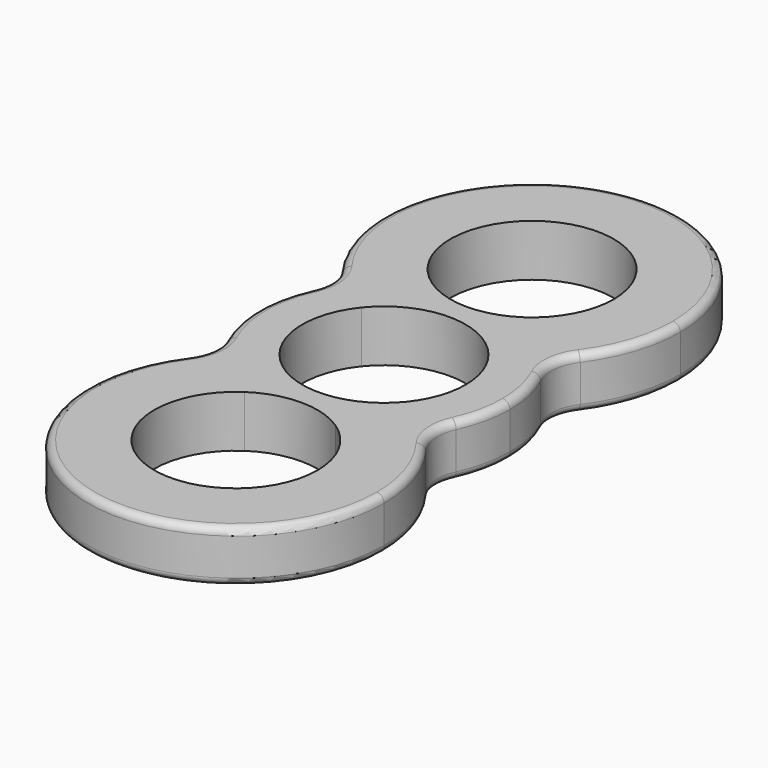
from build123d import *

# Parameters (mm, degrees)
F1_DEPTH = 7
F2_R     = 1


# Not quite as in the source:
# - a feature names something its author has since deleted; it is built from what else it names


with BuildPart() as f1:
    # F0 (on Top) → F1 (new body)
    with BuildSketch(Plane.XY):
        with BuildLine():
            ThreePointArc((8.5900351571, 6.911), (10.3984557172, 3.6637062787), (11.025, 0))
            ThreePointArc((11.025, 0), (10.3984557172, -3.6637062787), (8.5900351571, -6.911))
            ThreePointArc((8.5900351571, -6.911), (11.2087291798, -8.4058740762), (13.5732787491, -10.277))
            ThreePointArc((13.5732787491, -10.277), (14.5991765239, -8.7586911022), (15.455952476, -7.1389185498))
            ThreePointArc((15.455952476, -7.1389185498), (16.628111978, -3.6546568989), (17.025, 0))
            ThreePointArc((17.025, 0), (16.628111978, 3.6546568989), (15.455952476, 7.1389185498))
            ThreePointArc((15.455952476, 7.1389185498), (14.5991765239, 8.7586911022), (13.5732787491, 10.277))
            ThreePointArc((13.5732787491, 10.277), (11.2087291798, 8.4058740762), (8.5900351571, 6.911))
        make_face()
        with BuildLine():
            ThreePointArc((-8.5900351571, -6.911), (-11.025, 0), (-8.5900351571, 6.911))
            ThreePointArc((-8.5900351571, 6.911), (-11.2087291798, 8.4058740762), (-13.5732787491, 10.277))
            ThreePointArc((-13.5732787491, 10.277), (-14.5991765239, 8.7586911022), (-15.455952476, 7.1389185498))
            ThreePointArc((-15.455952476, 7.1389185498), (-17.025, 0), (-15.455952476, -7.1389185498))
            ThreePointArc((-15.455952476, -7.1389185498), (-14.5991765239, -8.7586911022), (-13.5732787491, -10.277))
            ThreePointArc((-13.5732787491, -10.277), (-11.2087291798, -8.4058740762), (-8.5900351571, -6.911))
        make_face()
        with BuildLine():
            ThreePointArc((6.1741937935, 15.866), (10.2615738659, 13.584944858), (13.5732787491, 10.277))
            ThreePointArc((13.5732787491, 10.277), (14.88595909, 11.6056412259), (16.0691422874, 13.0508037447))
            ThreePointArc((16.0691422874, 13.0508037447), (19.0103287623, 18.7065092876), (20.025, 25))
            ThreePointArc((20.025, 25), (-6.2934907124, 44.0103287623), (-16.0691422874, 13.0508037447))
            ThreePointArc((-16.0691422874, 13.0508037447), (-14.88595909, 11.6056412259), (-13.5732787491, 10.277))
            ThreePointArc((-13.5732787491, 10.277), (-10.2615738659, 13.584944858), (-6.1741937935, 15.866))
            ThreePointArc((-6.1741937935, 15.866), (-5.1710800819, 34.737071212), (11.025, 25))
            ThreePointArc((11.025, 25), (9.737071212, 19.8289199181), (6.1741937935, 15.866))
        make_face()
        with BuildLine():
            ThreePointArc((16.0691422874, 13.0508037447), (14.88595909, 11.6056412259), (13.5732787491, 10.277))
            ThreePointArc((13.5732787491, 10.277), (14.5991765239, 8.7586911022), (15.455952476, 7.1389185498))
            ThreePointArc((15.455952476, 7.1389185498), (14.9507513772, 10.1790618755), (16.0691422874, 13.0508037447))
        make_face()
        with BuildLine():
            ThreePointArc((16.0691422874, -13.0508037447), (14.88595909, -11.6056412259), (13.5732787491, -10.277))
            ThreePointArc((13.5732787491, -10.277), (10.2615738659, -13.584944858), (6.1741937935, -15.866))
            ThreePointArc((6.1741937935, -15.866), (9.737071212, -19.8289199181), (11.025, -25))
            ThreePointArc((11.025, -25), (-5.1710800819, -34.737071212), (-6.1741937935, -15.866))
            ThreePointArc((-6.1741937935, -15.866), (-10.2615738659, -13.584944858), (-13.5732787491, -10.277))
            ThreePointArc((-13.5732787491, -10.277), (-14.88595909, -11.6056412259), (-16.0691422874, -13.0508037447))
            ThreePointArc((-16.0691422874, -13.0508037447), (-6.2934907124, -44.0103287623), (20.025, -25))
            ThreePointArc((20.025, -25), (19.0103287623, -18.7065092876), (16.0691422874, -13.0508037447))
        make_face()
        with BuildLine():
            ThreePointArc((15.455952476, -7.1389185498), (14.5991765239, -8.7586911022), (13.5732787491, -10.277))
            ThreePointArc((13.5732787491, -10.277), (14.88595909, -11.6056412259), (16.0691422874, -13.0508037447))
            ThreePointArc((16.0691422874, -13.0508037447), (14.9507513772, -10.1790618755), (15.455952476, -7.1389185498))
        make_face()
        with BuildLine():
            ThreePointArc((-15.455952476, 7.1389185498), (-14.5991765239, 8.7586911022), (-13.5732787491, 10.277))
            ThreePointArc((-13.5732787491, 10.277), (-14.88595909, 11.6056412259), (-16.0691422874, 13.0508037447))
            ThreePointArc((-16.0691422874, 13.0508037447), (-14.9507513772, 10.1790618755), (-15.455952476, 7.1389185498))
        make_face()
        with BuildLine():
            ThreePointArc((-16.0691422874, -13.0508037447), (-14.88595909, -11.6056412259), (-13.5732787491, -10.277))
            ThreePointArc((-13.5732787491, -10.277), (-14.5991765239, -8.7586911022), (-15.455952476, -7.1389185498))
            ThreePointArc((-15.455952476, -7.1389185498), (-14.9507513772, -10.1790618755), (-16.0691422874, -13.0508037447))
        make_face()
        with BuildLine():
            ThreePointArc((-8.5900351571, 6.911), (0, 11.025), (8.5900351571, 6.911))
            ThreePointArc((8.5900351571, 6.911), (11.2087291798, 8.4058740762), (13.5732787491, 10.277))
            ThreePointArc((13.5732787491, 10.277), (10.2615738659, 13.584944858), (6.1741937935, 15.866))
            ThreePointArc((6.1741937935, 15.866), (0, 13.975), (-6.1741937935, 15.866))
            ThreePointArc((-6.1741937935, 15.866), (-10.2615738659, 13.584944858), (-13.5732787491, 10.277))
            ThreePointArc((-13.5732787491, 10.277), (-11.2087291798, 8.4058740762), (-8.5900351571, 6.911))
        make_face()
        with BuildLine():
            ThreePointArc((13.5732787491, -10.277), (11.2087291798, -8.4058740762), (8.5900351571, -6.911))
            ThreePointArc((8.5900351571, -6.911), (0, -11.025), (-8.5900351571, -6.911))
            ThreePointArc((-8.5900351571, -6.911), (-11.2087291798, -8.4058740762), (-13.5732787491, -10.277))
            ThreePointArc((-13.5732787491, -10.277), (-10.2615738659, -13.584944858), (-6.1741937935, -15.866))
            ThreePointArc((-6.1741937935, -15.866), (0, -13.975), (6.1741937935, -15.866))
            ThreePointArc((6.1741937935, -15.866), (10.2615738659, -13.584944858), (13.5732787491, -10.277))
        make_face()
    extrude(amount=F1_DEPTH)

    # F2
    f2_edges = [f1.edges().sort_by_distance(p)[0] for p in [
        (16.069142, 13.050804, 3.5),
        (-16.069142, 13.050804, 3.5),
        (0, 45.025, 0),
        (0, 45.025, 7),
        (-15.455952, 7.138919, 3.5),
        (-14.950751, 10.179062, 0),
        (-14.950751, 10.179062, 7),
        (-15.455952, -7.138919, 3.5),
        (-16.069142, -13.050804, 3.5),
        (-14.950751, -10.179062, 0),
        (-14.950751, -10.179062, 7),
        (16.069142, -13.050804, 3.5),
        (0, -45.025, 0),
        (0, -45.025, 7),
    ]]
    fillet(f2_edges, radius=F2_R)


solid = f1.part
